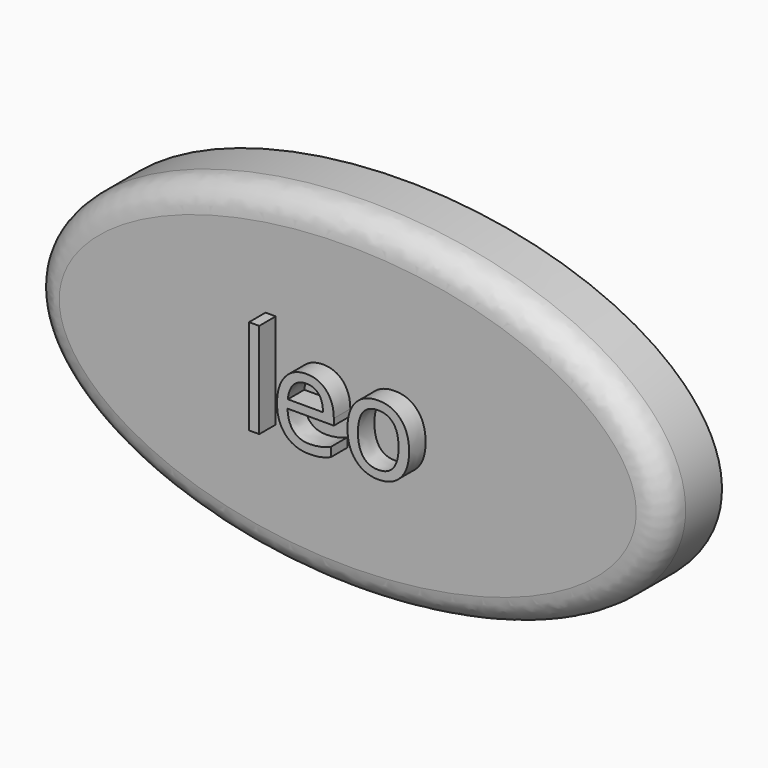
from build123d import *

# Parameters (mm, degrees)
F1_DEPTH     = 13.462
F2_R         = 5.08
F3_TEXT_SIZE = 23.1794482614
F4_DEPTH     = 3.81


# Not quite as in the source:
# - Text() gives the source's letters only with a copy of the font that has no kerning and outlines rounded to 1/6400 em; it was checked with that copy


with BuildPart() as f1:
    # F0 (on Front) → F1 (new body)
    with BuildSketch(Plane.XZ):
        with BuildLine():
            add(Edge.make_bspline(
                [(-58.3782307804, 0), (-58.3782307804, -53.9722503725), (29.1891153902, -26.9861251863), (116.7564615607, 0), (29.1891153902, 26.9861251863), (-58.3782307804, 53.9722503725), (-58.3782307804, 0)],
                knots=[0, 0, 0, 2.0943951024, 2.0943951024, 4.1887902048, 4.1887902048, 6.2831853072, 6.2831853072, 6.2831853072], degree=2, weights=[1, 0.5, 1, 0.5, 1, 0.5, 1]))
        make_face()
    extrude(amount=F1_DEPTH)

    # F2
    f2_edges = [f1.edges().sort_by_distance(p)[0] for p in [
        (58.378231, -13.462, -3e-06),
    ]]
    fillet(f2_edges, radius=F2_R)

    # F3 (on face) → F4 (join)
    with BuildSketch(Plane.XZ.offset(13.462)):
        with Locations((-17.1800609678, -7.362883538)):
            Text('leo', F3_TEXT_SIZE, font='Open Sans', text_align=(TextAlign.LEFT, TextAlign.BOTTOM))
    extrude(amount=F4_DEPTH)


solid = f1.part
